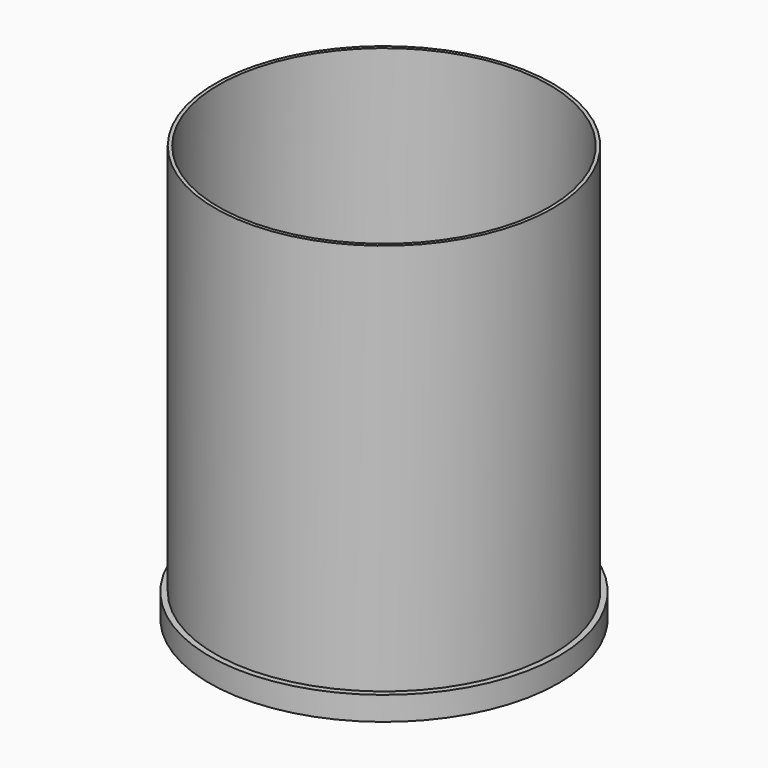
from build123d import *

# Parameters (mm, degrees)
F0_R      = 75
F1_DEPTH  = 5
F0_R_2    = 79
F2_DEPTH  = 30
F3_R      = 142.5
F3_R_2    = 79
F3_R_3    = 75
F4_DEPTH  = 5
F3_R_4    = 145.5
F5_DEPTH  = 158
F6_DEPTH  = 180
F7_R      = 150.5
F7_R_2    = 145.5
F7_R_3    = 142.5
F8_DEPTH  = 7.5
F9_R      = 150.5
F9_R_2    = 147
F10_DEPTH = 13
F11_R     = 7
F11_R_2   = 4
F12_DEPTH = 7
F13_D     = 5.5
F13_DEPTH = 12
F13_TIP   = 1.6523667023


with BuildPart() as f1:
    # F0 (on Top) → F1 (new body)
    with BuildSketch(Plane.XY):
        Circle(F0_R)
        with BuildLine():
            ThreePointArc((-27.2772727273, 3.4929060339), (0, 27.5), (27.2772727273, 3.4929060339))
            ThreePointArc((27.2772727273, 3.4929060339), (31, 0), (27.2772727273, -3.4929060339))
            ThreePointArc((27.2772727273, -3.4929060339), (0, -27.5), (-27.2772727273, -3.4929060339))
            ThreePointArc((-27.2772727273, -3.4929060339), (-31, 0), (-27.2772727273, 3.4929060339))
        make_face(mode=Mode.SUBTRACT)
    extrude(amount=F1_DEPTH)

    # F0 (on Top) → F2 (join)
    with BuildSketch(Plane.XY):
        Circle(F0_R_2)
        Circle(F0_R, mode=Mode.SUBTRACT)
    extrude(amount=F2_DEPTH)

    # F3 (on face) → F4 (join)
    with BuildSketch(Plane.XY.offset(30)):
        Circle(F3_R)
        Circle(F3_R_2, mode=Mode.SUBTRACT)
        Circle(F3_R_2)
        Circle(F3_R_3, mode=Mode.SUBTRACT)
    extrude(amount=F4_DEPTH)

    # F3 (on face) → F5 (join)
    with BuildSketch(Plane.XY.offset(30)):
        Circle(F3_R_4)
        Circle(F3_R, mode=Mode.SUBTRACT)
    extrude(amount=F5_DEPTH)

    # F3 (on face) → F6 (join)
    with BuildSketch(Plane.XY.offset(30)):
        Circle(F3_R_4)
        Circle(F3_R, mode=Mode.SUBTRACT)
    extrude(amount=-F6_DEPTH)

    # F7 (on face) → F8 (join)
    with BuildSketch(Plane(origin=(0, 0, -150), x_dir=(1, 0, 0), z_dir=(0, 0, -1))):
        Circle(F7_R)
        Circle(F7_R_2, mode=Mode.SUBTRACT)
        Circle(F7_R_2)
        Circle(F7_R_3, mode=Mode.SUBTRACT)
    extrude(amount=F8_DEPTH)

    # F9 (on face) → F10 (join)
    with BuildSketch(Plane(origin=(0, 0, -157.5), x_dir=(1, 0, 0), z_dir=(0, 0, -1))):
        Circle(F9_R)
        Circle(F9_R_2, mode=Mode.SUBTRACT)
    extrude(amount=F10_DEPTH)

    # F11 (on face) → F12 (join)
    with BuildSketch(Plane.XY.offset(35)):
        with Locations((0, 83.2192561637)):
            Circle(F11_R)
        with Locations((0, 83.2192561637)):
            Circle(F11_R_2, mode=Mode.SUBTRACT)
        with Locations((-65, -51.9658021822)):
            Circle(F11_R)
        with Locations((-65, -51.9658021822)):
            Circle(F11_R_2, mode=Mode.SUBTRACT)
        with Locations((65, -51.9658021822)):
            Circle(F11_R)
        with Locations((65, -51.9658021822)):
            Circle(F11_R_2, mode=Mode.SUBTRACT)
    extrude(amount=F12_DEPTH)

    # F13
    with Locations(Plane.XY.offset(35)):
        with Locations((0, 83.2192561637), (-65, -51.9658021822), (65, -51.9658021822)):
            Hole(F13_D / 2, depth=F13_DEPTH)
            with Locations((0, 0, -(F13_DEPTH + F13_TIP / 2))):  # 118° drill point
                Cone(0, F13_D / 2, F13_TIP, mode=Mode.SUBTRACT)


solid = f1.part
